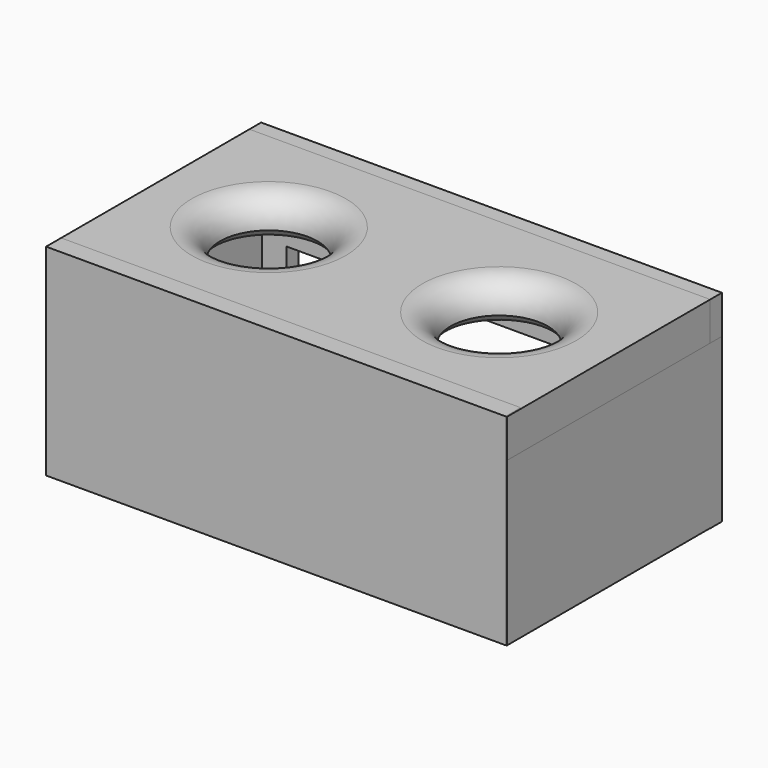
from build123d import *

# Parameters (mm, degrees)
F0_W      = 60
F0_H      = 70
F0_R      = 12.6947859899
F0_R_2    = 12.7
F1_DEPTH  = 10
F2_R      = 7.3585229381
F4_W      = 69.4058109075
F4_H      = 42.471062392
F5_DEPTH  = 3.302
F6_W      = 120
F6_H      = 52.471062392
F7_DEPTH  = 3.81
F8_W      = 3.5209719837
F8_H      = 70
F9_DEPTH  = 42.418
F10_R     = 2.2359129528
F11_DEPTH = 17.6784
F12_W     = 4.9080215394
F12_H     = 52.471062392
F13_DEPTH = 119.634
F14_W     = 100.1165024936
F14_H     = 14.1438832507
F15_DEPTH = 16.256


# Not quite as in the source:
# - a fillet or chamfer that OpenCascade refuses, or shapes differently, is made with other operations: its cross-section is extruded or revolved along the edge and cut away or added


with BuildPart() as f1:
    # F0 (on Top) → F1 (new body)
    with BuildSketch(Plane.XY):
        with Locations((19.8352524638, -15.612911582)):
            Rectangle(F0_W, F0_H)
        with Locations((19.8352524638, -15.612911582)):
            Circle(F0_R, mode=Mode.SUBTRACT)
        with Locations((-40.1647475362, -15.612911582)):
            Rectangle(F0_W, F0_H)
        with Locations((-40.1647475362, -15.612911582)):
            Circle(F0_R_2, mode=Mode.SUBTRACT)
    extrude(amount=F1_DEPTH)

    # F2
    f2_edges = [f1.edges().sort_by_distance(p)[0] for p in [
        (-52.864748, -15.612912, 10),
        (7.140466, -15.612912, 10),
    ]]
    fillet(f2_edges, radius=F2_R)

    # F3: fillet of radius 5.08 on 2 edges, made by hand

    # F3_s1 → F3_t2 (revolve, cut)
    with BuildSketch(Plane.XZ.offset(15.612911582)):
        with BuildLine():
            ThreePointArc((-23.0082908854, 0), (-25.5985325222, 0.7099830363), (-27.4647475362, 2.6414770619))
            Line((-27.4647475362, 2.6414770619), (-27.4647475362, 0))
            Line((-27.4647475362, 0), (-23.0082908854, 0))
        make_face()
    revolve(axis=Axis((-40.1647475362, -15.612911582, 0), (0, 0, 1)), mode=Mode.SUBTRACT)

    # F3_s3 → F3_t4 (revolve, cut)
    with BuildSketch(Plane.XZ.offset(15.612911582)):
        with BuildLine():
            ThreePointArc((32.5300384537, 2.6414770619), (34.3962534676, 0.7099830363), (36.9864951045, 0))
            Line((36.9864951045, 0), (32.5300384537, 0))
            Line((32.5300384537, 0), (32.5300384537, 2.6414770619))
        make_face()
    revolve(axis=Axis((19.8352524638, -15.612911582, 0), (0, 0, 1)), mode=Mode.SUBTRACT)

    # F4 (on face) → F5 (join)
    with BuildSketch(Plane(origin=(-70.1647475362, 0, 0), x_dir=(0, -1, 0), z_dir=(-1, 0, 0))):
        with Locations((15.4800685123, -21.235531196)):
            Rectangle(F4_W, F4_H)
    extrude(amount=-F5_DEPTH)

    # F10 (on face) → F11 (join)
    with BuildSketch(Plane.XZ.offset(50.612911582)):
        with Locations((-63.7861341238, 5.1306239329)):
            Circle(F10_R)
    extrude(amount=-F11_DEPTH)


with BuildPart() as f7:
    # F6 (on face) → F7 (new body)
    with BuildSketch(Plane(origin=(0, 19.387088418, 0), x_dir=(-1, 0, 0), z_dir=(0, 1, 0))):
        with Locations((10.1647475362, -16.235531196)):
            Rectangle(F6_W, F6_H)
    extrude(amount=-F7_DEPTH)

    # F14 (on face) → F15 (cut)
    with BuildSketch(Plane(origin=(0, 19.387088418, 0), x_dir=(-1, 0, 0), z_dir=(0, 1, 0))):
        with Locations((10.3999134153, -20.7998272963)):
            Rectangle(F14_W, F14_H)
    extrude(amount=-F15_DEPTH, mode=Mode.SUBTRACT)


with BuildPart() as f9:
    # F8 (on face) → F9 (new body)
    with BuildSketch(Plane(origin=(0, 0, 0), x_dir=(1, 0, 0), z_dir=(0, 0, -1))):
        with Locations((48.074766472, 15.612911582)):
            Rectangle(F8_W, F8_H)
    extrude(amount=F9_DEPTH)


with BuildPart() as f13:
    # F12 (on face) → F13 (new body)
    with BuildSketch(Plane(origin=(-70.1647475362, 0, 0), x_dir=(0, -1, 0), z_dir=(-1, 0, 0))):
        with Locations((48.1589008123, -16.235531196)):
            Rectangle(F12_W, F12_H)
    extrude(amount=-F13_DEPTH)


solid = Compound([f1.part, f7.part, f9.part, f13.part])
